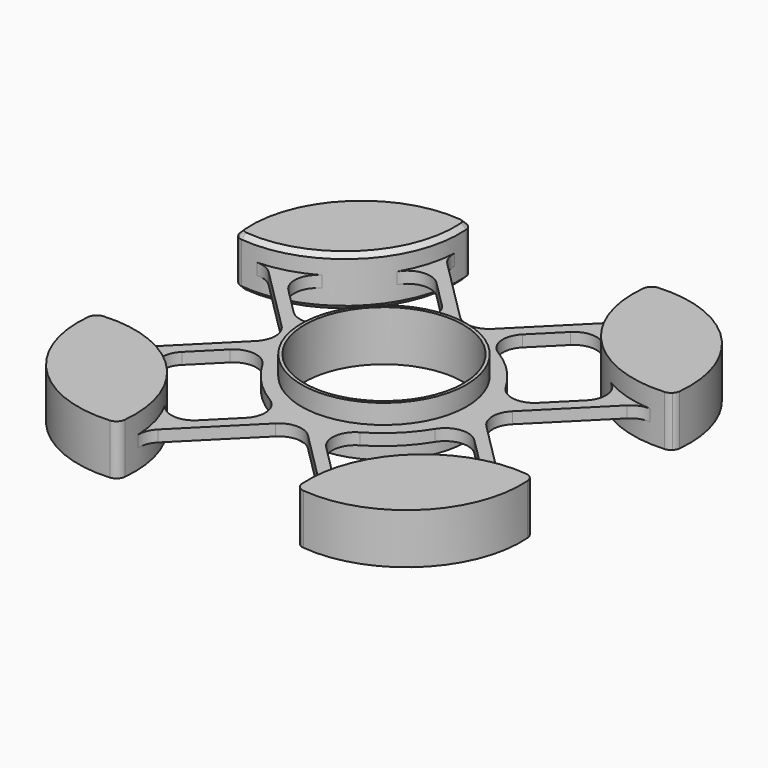
from build123d import *

# Parameters (mm, degrees)
F0_R     = 11.43
F1_DEPTH = 0.79375
F2_R     = 11.43
F2_R_2   = 10.9855
F3_DEPTH = 3.4798
F5_DEPTH = 3.4798
F6_R     = 3.175
F7_SIZE  = 0.635


# Not quite as in the source:
# - a feature names something its author has since deleted; it is built from what else it names


with BuildPart() as f1:
    # F0 (on Top) → F1 (new body, symmetric)
    with BuildSketch(Plane.XY):
        Polygon((-14.3684097937, 28.0844097937), (-28.2927262655, 14.5767262655), (-13.716, 0), (-28.0844097937, -14.3684097937), (-14.5767262655, -28.2927262655), (0, -13.716), (14.3684097937, -28.0844097937), (28.2927262655, -14.5767262655), (13.716, 0), (28.0844097937, 14.3684097937), (14.5767262655, 28.2927262655), (0, 13.716), align=None)
        with BuildLine():
            ThreePointArc((-13.0320412256, -24.4131746341), (-20.1396997698, -20.0947125947), (-24.2403197525, -12.8591863439))
            Line((-24.2403197525, -12.8591863439), (-13.5538149684, -2.1726815599))
            ThreePointArc((-13.5538149684, -2.1726815599), (-9.4531949857, -9.4082078106), (-2.3455364415, -13.72666985))
            Line((-2.3455364415, -13.72666985), (-13.0320412256, -24.4131746341))
        make_face(mode=Mode.SUBTRACT)
        with BuildLine():
            ThreePointArc((24.4131746341, -13.0320412256), (20.0947125947, -20.1396997698), (12.8591863439, -24.2403197525))
            Line((12.8591863439, -24.2403197525), (2.1726815599, -13.5538149684))
            ThreePointArc((2.1726815599, -13.5538149684), (9.4082078106, -9.4531949857), (13.72666985, -2.3455364415))
            Line((13.72666985, -2.3455364415), (24.4131746341, -13.0320412256))
        make_face(mode=Mode.SUBTRACT)
        Circle(F0_R, mode=Mode.SUBTRACT)
        with BuildLine():
            ThreePointArc((-2.1726815599, 13.5538149684), (-9.4082078106, 9.4531949857), (-13.72666985, 2.3455364415))
            Line((-13.72666985, 2.3455364415), (-24.4131746341, 13.0320412256))
            ThreePointArc((-24.4131746341, 13.0320412256), (-20.0947125947, 20.1396997698), (-12.8591863439, 24.2403197525))
            Line((-12.8591863439, 24.2403197525), (-2.1726815599, 13.5538149684))
        make_face(mode=Mode.SUBTRACT)
        with BuildLine():
            ThreePointArc((13.0320412256, 24.4131746341), (20.1396997698, 20.0947125947), (24.2403197525, 12.8591863439))
            Line((24.2403197525, 12.8591863439), (13.5538149684, 2.1726815599))
            ThreePointArc((13.5538149684, 2.1726815599), (9.4531949857, 9.4082078106), (2.3455364415, 13.72666985))
            Line((2.3455364415, 13.72666985), (13.0320412256, 24.4131746341))
        make_face(mode=Mode.SUBTRACT)
    extrude(amount=F1_DEPTH, both=True)

    # F2 (on Top) → F3 (join, symmetric)
    with BuildSketch(Plane.XY):
        Circle(F2_R)
        Circle(F2_R_2, mode=Mode.SUBTRACT)
    extrude(amount=F3_DEPTH, both=True)

    # F4 (on Top) → F5 (join, symmetric)
    with BuildSketch(Plane.XY):
        with BuildLine():
            ThreePointArc((-13.1605476158, 30.3918186243), (-25.856934394, 25.9965462925), (-30.6357520227, 13.4394941638))
            ThreePointArc((-30.6357520227, 13.4394941638), (-30.5278746276, 13.0126091951), (-30.2807216131, 12.6482142222))
            Line((-30.2807216131, 12.6482142222), (-12.3804144461, 30.0129218371))
            ThreePointArc((-12.3804144461, 30.0129218371), (-12.7371356357, 30.2710270515), (-13.1605476158, 30.3918186243))
        make_face()
        with BuildLine():
            Line((-12.3804144461, 30.0129218371), (-30.2807216131, 12.6482142222))
            ThreePointArc((-30.2807216131, 12.6482142222), (-29.9240004235, 12.3901090077), (-29.5005884435, 12.2693174349))
            ThreePointArc((-29.5005884435, 12.2693174349), (-16.8042016652, 16.6645897667), (-12.0253840365, 29.2216418954))
            ThreePointArc((-12.0253840365, 29.2216418954), (-12.1332614316, 29.6485268641), (-12.3804144461, 30.0129218371))
        make_face()
        with BuildLine():
            ThreePointArc((-30.3918186243, -13.1605476158), (-25.9965462925, -25.856934394), (-13.4394941638, -30.6357520227))
            ThreePointArc((-13.4394941638, -30.6357520227), (-13.0126091951, -30.5278746276), (-12.6482142222, -30.2807216131))
            Line((-12.6482142222, -30.2807216131), (-30.0129218371, -12.3804144461))
            ThreePointArc((-30.0129218371, -12.3804144461), (-30.2710270515, -12.7371356357), (-30.3918186243, -13.1605476158))
        make_face()
        with BuildLine():
            Line((-30.0129218371, -12.3804144461), (-12.6482142222, -30.2807216131))
            ThreePointArc((-12.6482142222, -30.2807216131), (-12.3901090077, -29.9240004235), (-12.2693174349, -29.5005884435))
            ThreePointArc((-12.2693174349, -29.5005884435), (-16.6645897667, -16.8042016652), (-29.2216418954, -12.0253840365))
            ThreePointArc((-29.2216418954, -12.0253840365), (-29.6485268641, -12.1332614316), (-30.0129218371, -12.3804144461))
        make_face()
        with BuildLine():
            ThreePointArc((13.1605476158, -30.3918186243), (25.856934394, -25.9965462925), (30.6357520227, -13.4394941638))
            ThreePointArc((30.6357520227, -13.4394941638), (30.5278746276, -13.0126091951), (30.2807216131, -12.6482142222))
            Line((30.2807216131, -12.6482142222), (12.3804144461, -30.0129218371))
            ThreePointArc((12.3804144461, -30.0129218371), (12.7371356357, -30.2710270515), (13.1605476158, -30.3918186243))
        make_face()
        with BuildLine():
            Line((12.3804144461, -30.0129218371), (30.2807216131, -12.6482142222))
            ThreePointArc((30.2807216131, -12.6482142222), (29.9240004235, -12.3901090077), (29.5005884435, -12.2693174349))
            ThreePointArc((29.5005884435, -12.2693174349), (16.8042016652, -16.6645897667), (12.0253840365, -29.2216418954))
            ThreePointArc((12.0253840365, -29.2216418954), (12.1332614316, -29.6485268641), (12.3804144461, -30.0129218371))
        make_face()
        with BuildLine():
            ThreePointArc((30.3918186243, 13.1605476158), (25.9965462925, 25.856934394), (13.4394941638, 30.6357520227))
            ThreePointArc((13.4394941638, 30.6357520227), (13.0126091951, 30.5278746276), (12.6482142222, 30.2807216131))
            Line((12.6482142222, 30.2807216131), (30.0129218371, 12.3804144461))
            ThreePointArc((30.0129218371, 12.3804144461), (30.2710270515, 12.7371356357), (30.3918186243, 13.1605476158))
        make_face()
        with BuildLine():
            Line((30.0129218371, 12.3804144461), (12.6482142222, 30.2807216131))
            ThreePointArc((12.6482142222, 30.2807216131), (12.3901090077, 29.9240004235), (12.2693174349, 29.5005884435))
            ThreePointArc((12.2693174349, 29.5005884435), (16.6645897667, 16.8042016652), (29.2216418954, 12.0253840365))
            ThreePointArc((29.2216418954, 12.0253840365), (29.6485268641, 12.1332614316), (30.0129218371, 12.3804144461))
        make_face()
    extrude(amount=F5_DEPTH, both=True)

    # F6
    f6_edges = [f1.edges().sort_by_distance(p)[0] for p in [
        (-26.008197, 12.292197, 0),
        (-12.533339, 23.914473, 0),
        (-24.032883, 12.65175, 0),
        (-12.136817, 25.852817, 0),
        (-2.172682, 13.553815, 0),
        (-13.72667, 2.345536, 0),
        (-13.716, 0, 0),
        (0, 13.716, 0),
        (2.345536, 13.72667, 0),
        (13.553815, 2.172682, 0),
        (13.716, 0, 0),
        (13.72667, -2.345536, 0),
        (2.172682, -13.553815, 0),
        (0, -13.716, 0),
        (-2.345536, -13.72667, 0),
        (-13.553815, -2.172682, 0),
        (12.292197, 26.008197, 0),
        (12.65175, 24.032883, 0),
        (25.852817, 12.136817, 0),
        (23.914473, 12.533339, 0),
        (26.008197, -12.292197, 0),
        (24.032883, -12.65175, 0),
        (12.136817, -25.852817, 0),
        (12.533339, -23.914473, 0),
        (-12.292197, -26.008197, 0),
        (-12.65175, -24.032883, 0),
        (-25.852817, -12.136817, 0),
        (-23.914473, -12.533339, 0),
    ]]
    fillet(f6_edges, radius=F6_R)

    # F7
    f7_edges = [f1.edges().sort_by_distance(p)[0] for p in [
        (-25.856934, 25.996546, 3.4798),
        (-30.280722, 12.648214, 3.4798),
        (-16.804202, 16.66459, 3.4798),
        (-12.380414, 30.012922, 3.4798),
        (-25.856934, 25.996546, -3.4798),
        (-30.280722, 12.648214, -3.4798),
        (-16.804202, 16.66459, -3.4798),
        (-12.380414, 30.012922, -3.4798),
    ]]
    chamfer(f7_edges, length=F7_SIZE)


solid = f1.part
